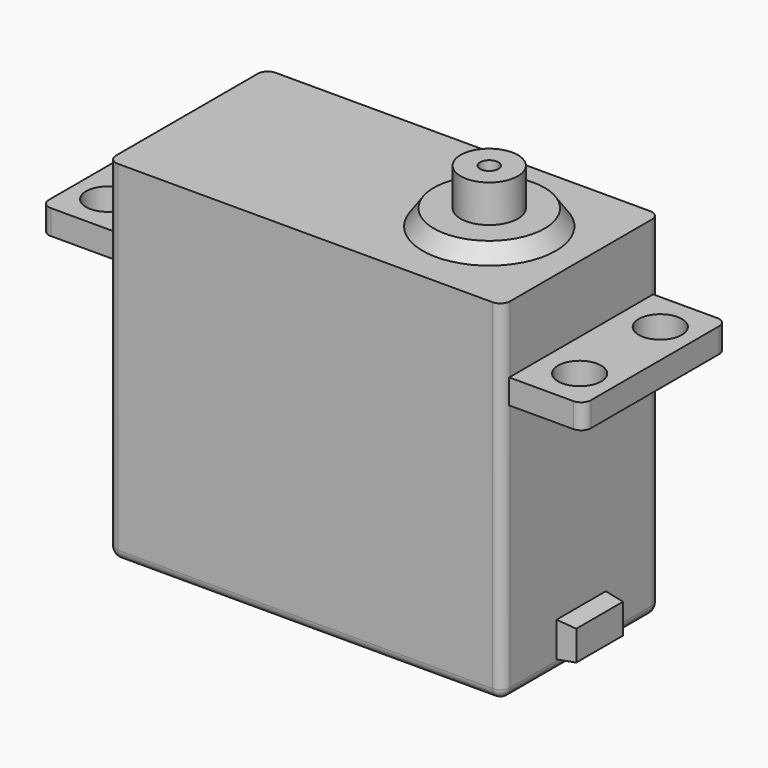
from build123d import *

# Parameters (mm, degrees)
F0_W           = 40.64
F0_H           = 20.32
F1_DEPTH       = 36.068
F2_W           = 6.35
F2_H           = 3.6068
F4_W           = 6.0198
F4_H           = 3.0734
F7_R           = 2.2225
F8_DEPTH       = 2.54
F9_R           = 6.858
F11_R          = 5.7023
F13_T1_DEPTH   = 38.608
F13_T3_DEPTH   = 18.288
F13_S7_W       = 1.016
F13_S7_H       = 1.016
F13_T8_DEPTH   = 1.016
F13_S13_W      = 1.016
F13_S13_H      = 1.016
F13_T14_DEPTH  = 1.016
F13_S19_W      = 1.016
F13_S19_H      = 1.016
F13_T20_DEPTH  = 1.016
F13_S25_W      = 1.016
F13_S25_H      = 1.016
F13_T26_DEPTH  = 1.016
F13_T32_DEPTH  = 37.592
F13_T38_DEPTH  = 37.592
F13_T44_DEPTH  = 37.592
F13_T51_DEPTH  = 37.592
F13_T57_DEPTH  = 37.592
F13_T63_DEPTH  = 37.592
F13_T69_DEPTH  = 37.592
F13_T75_DEPTH  = 37.592
F13_T82_DEPTH  = 37.592
F13_T88_DEPTH  = 37.592
F13_T94_DEPTH  = 37.592
F13_T100_DEPTH = 37.592
F13_T106_DEPTH = 37.592
F13_T113_DEPTH = 37.592
F13_T119_DEPTH = 37.592
F13_T125_DEPTH = 37.592
F13_T131_DEPTH = 37.592
F13_T137_DEPTH = 37.592
F13_T144_DEPTH = 37.592
F13_T150_DEPTH = 37.592
F14_R          = 2.95275
F14_R_2        = 0.9398
F15_DEPTH      = 3.8608


# Not quite as in the source:
# - a fillet or chamfer that OpenCascade refuses, or shapes differently, is made with other operations: its cross-section is extruded or revolved along the edge and cut away or added


with BuildPart() as f1:
    # F0 (on Top) → F1 (new body)
    with BuildSketch(Plane.XY):
        Rectangle(F0_W, F0_H)
    extrude(amount=F1_DEPTH)

    # F2 (on face) → F5 section 0
    with BuildSketch(Plane.YZ.offset(20.32)):
        with Locations((0, 2.9464)):
            Rectangle(F2_W, F2_H)
    # F4 (on offset) → F5 section 1
    with BuildSketch(Plane.YZ.offset(22.225)):
        with Locations((0, 2.9464)):
            Rectangle(F4_W, F4_H)
    loft()

    # F7 (on offset) → F8 (join)
    with BuildSketch(Plane.XY.offset(29.21)):
        with BuildLine():
            ThreePointArc((-27.94, -8.255), (-27.6424204897, -8.9734204897), (-26.924, -9.271))
            Line((-26.924, -9.271), (-20.32, -9.271))
            Line((-20.32, -9.271), (-20.32, 9.271))
            Line((-20.32, 9.271), (-26.924, 9.271))
            ThreePointArc((-26.924, 9.271), (-27.6424204897, 8.9734204897), (-27.94, 8.255))
            Line((-27.94, 8.255), (-27.94, -8.255))
        make_face()
        with Locations((-24.3205, -5.1943)):
            Circle(F7_R, mode=Mode.SUBTRACT)
        with Locations((-24.3205, 5.1943)):
            Circle(F7_R, mode=Mode.SUBTRACT)
        with BuildLine():
            ThreePointArc((27.94, 8.255), (27.6424204897, 8.9734204897), (26.924, 9.271))
            Line((26.924, 9.271), (20.32, 9.271))
            Line((20.32, 9.271), (20.32, -9.271))
            Line((20.32, -9.271), (26.924, -9.271))
            ThreePointArc((26.924, -9.271), (27.6424204897, -8.9734204897), (27.94, -8.255))
            Line((27.94, -8.255), (27.94, 8.255))
        make_face()
        with Locations((24.3205, -5.1943)):
            Circle(F7_R, mode=Mode.SUBTRACT)
        with Locations((24.3205, 5.1943)):
            Circle(F7_R, mode=Mode.SUBTRACT)
    extrude(amount=-F8_DEPTH)

    # F9 (on face) → F12 section 0
    with BuildSketch(Plane.XY.offset(36.068)):
        with Locations((10.8458, 0)):
            Circle(F9_R)
    # F11 (on offset) → F12 section 1
    with BuildSketch(Plane.XY.offset(37.719)):
        with Locations((10.8458, 0)):
            Circle(F11_R)
    loft()

    # F13: fillet of radius 1.016 on 8 edges, made by hand

    # F13_s2 → F13_t1 (cut)
    with BuildSketch(Plane.YZ.offset(-19.304)):
        with BuildLine():
            ThreePointArc((-10.16, 1.016), (-9.8624204897, 0.2975795103), (-9.144, 0))
            Line((-9.144, 0), (-10.16, 0))
            Line((-10.16, 0), (-10.16, 1.016))
        make_face()
        with BuildLine():
            ThreePointArc((9.144, 0), (9.8624204897, 0.2975795103), (10.16, 1.016))
            Line((10.16, 1.016), (10.16, 0))
            Line((10.16, 0), (9.144, 0))
        make_face()
    extrude(amount=F13_T1_DEPTH, mode=Mode.SUBTRACT)

    # F13_s4 → F13_t3 (cut)
    with BuildSketch(Plane.XZ.offset(-9.144)):
        with BuildLine():
            ThreePointArc((20.32, 1.016), (20.0224204897, 0.2975795103), (19.304, 0))
            Line((19.304, 0), (20.32, 0))
            Line((20.32, 0), (20.32, 1.016))
        make_face()
        with BuildLine():
            ThreePointArc((-19.304, 0), (-20.0224204897, 0.2975795103), (-20.32, 1.016))
            Line((-20.32, 1.016), (-20.32, 0))
            Line((-20.32, 0), (-19.304, 0))
        make_face()
    extrude(amount=F13_T3_DEPTH, mode=Mode.SUBTRACT)


with BuildPart() as f13_tool6:
    # F13_s7 → F13_t8 (new body)
    with BuildSketch(Plane.YZ.offset(19.304)):
        with Locations((-9.652, 0.508)):
            Rectangle(F13_S7_W, F13_S7_H)
    extrude(amount=F13_T8_DEPTH)

    # F13_s9 → F13_t10 (revolve, cut)
    with BuildSketch(Plane(origin=(19.304, -9.144, 1.016), x_dir=(0, 0.7071067812, 0.7071067812), z_dir=(0, 0.7071067812, -0.7071067812))):
        with BuildLine():
            ThreePointArc((0, -1.016), (1.016, 0), (0, 1.016))
            Line((0, 1.016), (0, -1.016))
        make_face()
    revolve(axis=Axis((19.304, -9.144, 1.016), (1, 0, 0)), mode=Mode.SUBTRACT)


with BuildPart() as f1_1:
    add(f1.part)

    # F13_t5: cut F13_tool6
    add(f13_tool6.part, mode=Mode.SUBTRACT)


with BuildPart() as f13_tool12:
    # F13_s13 → F13_t14 (new body)
    with BuildSketch(Plane.YZ.offset(19.304)):
        with Locations((9.652, 0.508)):
            Rectangle(F13_S13_W, F13_S13_H)
    extrude(amount=F13_T14_DEPTH)

    # F13_s15 → F13_t16 (revolve, cut)
    with BuildSketch(Plane(origin=(19.304, 9.144, 1.016), x_dir=(0, -0.7071067812, 0.7071067812), z_dir=(0, 0.7071067812, 0.7071067812))):
        with BuildLine():
            ThreePointArc((0, -1.016), (1.016, 0), (0, 1.016))
            Line((0, 1.016), (0, -1.016))
        make_face()
    revolve(axis=Axis((19.304, 9.144, 1.016), (1, 0, 0)), mode=Mode.SUBTRACT)


with BuildPart() as f1_2:
    add(f1_1.part)

    # F13_t11: cut F13_tool12
    add(f13_tool12.part, mode=Mode.SUBTRACT)


with BuildPart() as f13_tool18:
    # F13_s19 → F13_t20 (new body)
    with BuildSketch(Plane.XY.offset(1.016)):
        with Locations((-19.812, 9.652)):
            Rectangle(F13_S19_W, F13_S19_H)
    extrude(amount=-F13_T20_DEPTH)

    # F13_s21 → F13_t22 (revolve, cut)
    with BuildSketch(Plane(origin=(-19.304, 9.144, 1.016), x_dir=(0.7071067812, -0.7071067812, 0), z_dir=(0.7071067812, 0.7071067812, 0))):
        with BuildLine():
            ThreePointArc((0, -1.016), (1.016, 0), (0, 1.016))
            Line((0, 1.016), (0, -1.016))
        make_face()
    revolve(axis=Axis((-19.304, 9.144, 1.016), (0, 0, -1)), mode=Mode.SUBTRACT)


with BuildPart() as f1_3:
    add(f1_2.part)

    # F13_t17: cut F13_tool18
    add(f13_tool18.part, mode=Mode.SUBTRACT)


with BuildPart() as f13_tool24:
    # F13_s25 → F13_t26 (new body)
    with BuildSketch(Plane.XZ.offset(9.144)):
        with Locations((-19.812, 0.508)):
            Rectangle(F13_S25_W, F13_S25_H)
    extrude(amount=F13_T26_DEPTH)

    # F13_s27 → F13_t28 (revolve, cut)
    with BuildSketch(Plane(origin=(-19.304, -9.144, 1.016), x_dir=(0.7071067812, 0, 0.7071067812), z_dir=(0.7071067812, 0, -0.7071067812))):
        with BuildLine():
            ThreePointArc((0, -1.016), (1.016, 0), (0, 1.016))
            Line((0, 1.016), (0, -1.016))
        make_face()
    revolve(axis=Axis((-19.304, -9.144, 1.016), (0, -1, 0)), mode=Mode.SUBTRACT)


with BuildPart() as f1_4:
    add(f1_3.part)

    # F13_t23: cut F13_tool24
    add(f13_tool24.part, mode=Mode.SUBTRACT)


with BuildPart() as f13_tool30:
    # F13_s31 → F13_t32 (new body)
    with BuildSketch(Plane.XY.offset(1.016)):
        with BuildLine():
            ThreePointArc((20.32, -9.144), (20.0224204897, -9.8624204897), (19.304, -10.16))
            Line((19.304, -10.16), (20.32, -10.16))
            Line((20.32, -10.16), (20.32, -9.144))
        make_face()
    extrude(amount=F13_T32_DEPTH)

    split(bisect_by=Plane.XY.offset(26.67), keep=Keep.BOTTOM)

    split(bisect_by=Plane.XZ.offset(9.271), keep=Keep.BOTTOM)


with BuildPart() as f1_5:
    add(f1_4.part)

    # F13_t29: cut F13_tool30
    add(f13_tool30.part, mode=Mode.SUBTRACT)


with BuildPart() as f13_tool36:
    # F13_s37 → F13_t38 (new body)
    with BuildSketch(Plane.XY.offset(1.016)):
        with BuildLine():
            ThreePointArc((20.32, -9.144), (20.0224204897, -9.8624204897), (19.304, -10.16))
            Line((19.304, -10.16), (20.32, -10.16))
            Line((20.32, -10.16), (20.32, -9.144))
        make_face()
    extrude(amount=F13_T38_DEPTH)

    split(bisect_by=Plane.XY.offset(26.67), keep=Keep.BOTTOM)

    split(bisect_by=Plane.XZ.offset(9.271), keep=Keep.TOP)


with BuildPart() as f1_6:
    add(f1_5.part)

    # F13_t35: cut F13_tool36
    add(f13_tool36.part, mode=Mode.SUBTRACT)


with BuildPart() as f13_tool42:
    # F13_s43 → F13_t44 (new body)
    with BuildSketch(Plane.XY.offset(1.016)):
        with BuildLine():
            ThreePointArc((20.32, -9.144), (20.0224204897, -9.8624204897), (19.304, -10.16))
            Line((19.304, -10.16), (20.32, -10.16))
            Line((20.32, -10.16), (20.32, -9.144))
        make_face()
    extrude(amount=F13_T44_DEPTH)

    split(bisect_by=Plane.XY.offset(26.67), keep=Keep.TOP)

    split(bisect_by=Plane.XZ.offset(9.271), keep=Keep.TOP)

    split(bisect_by=Plane.XY.offset(29.21), keep=Keep.BOTTOM)


with BuildPart() as f1_7:
    add(f1_6.part)

    # F13_t41: cut F13_tool42
    add(f13_tool42.part, mode=Mode.SUBTRACT)


with BuildPart() as f13_tool49:
    # F13_s50 → F13_t51 (new body)
    with BuildSketch(Plane.XY.offset(1.016)):
        with BuildLine():
            ThreePointArc((20.32, -9.144), (20.0224204897, -9.8624204897), (19.304, -10.16))
            Line((19.304, -10.16), (20.32, -10.16))
            Line((20.32, -10.16), (20.32, -9.144))
        make_face()
    extrude(amount=F13_T51_DEPTH)

    split(bisect_by=Plane.XZ.offset(9.271), keep=Keep.BOTTOM)

    split(bisect_by=Plane.XY.offset(29.21), keep=Keep.TOP)


with BuildPart() as f1_8:
    add(f1_7.part)

    # F13_t48: cut F13_tool49
    add(f13_tool49.part, mode=Mode.SUBTRACT)


with BuildPart() as f13_tool55:
    # F13_s56 → F13_t57 (new body)
    with BuildSketch(Plane.XY.offset(1.016)):
        with BuildLine():
            ThreePointArc((20.32, -9.144), (20.0224204897, -9.8624204897), (19.304, -10.16))
            Line((19.304, -10.16), (20.32, -10.16))
            Line((20.32, -10.16), (20.32, -9.144))
        make_face()
    extrude(amount=F13_T57_DEPTH)

    split(bisect_by=Plane.XZ.offset(9.271), keep=Keep.TOP)

    split(bisect_by=Plane.XY.offset(29.21), keep=Keep.TOP)


with BuildPart() as f1_9:
    add(f1_8.part)

    # F13_t54: cut F13_tool55
    add(f13_tool55.part, mode=Mode.SUBTRACT)


with BuildPart() as f13_tool61:
    # F13_s62 → F13_t63 (new body)
    with BuildSketch(Plane.XY.offset(1.016)):
        with BuildLine():
            ThreePointArc((20.32, 9.144), (20.0224204897, 9.8624204897), (19.304, 10.16))
            Line((19.304, 10.16), (20.32, 10.16))
            Line((20.32, 10.16), (20.32, 9.144))
        make_face()
    extrude(amount=F13_T63_DEPTH)

    split(bisect_by=Plane.XZ.offset(-9.271), keep=Keep.TOP)

    split(bisect_by=Plane.XY.offset(26.67), keep=Keep.BOTTOM)


with BuildPart() as f1_10:
    add(f1_9.part)

    # F13_t60: cut F13_tool61
    add(f13_tool61.part, mode=Mode.SUBTRACT)


with BuildPart() as f13_tool67:
    # F13_s68 → F13_t69 (new body)
    with BuildSketch(Plane.XY.offset(1.016)):
        with BuildLine():
            ThreePointArc((20.32, 9.144), (20.0224204897, 9.8624204897), (19.304, 10.16))
            Line((19.304, 10.16), (20.32, 10.16))
            Line((20.32, 10.16), (20.32, 9.144))
        make_face()
    extrude(amount=F13_T69_DEPTH)

    split(bisect_by=Plane.XZ.offset(-9.271), keep=Keep.BOTTOM)

    split(bisect_by=Plane.XY.offset(26.67), keep=Keep.BOTTOM)


with BuildPart() as f1_11:
    add(f1_10.part)

    # F13_t66: cut F13_tool67
    add(f13_tool67.part, mode=Mode.SUBTRACT)


with BuildPart() as f13_tool73:
    # F13_s74 → F13_t75 (new body)
    with BuildSketch(Plane.XY.offset(1.016)):
        with BuildLine():
            ThreePointArc((20.32, 9.144), (20.0224204897, 9.8624204897), (19.304, 10.16))
            Line((19.304, 10.16), (20.32, 10.16))
            Line((20.32, 10.16), (20.32, 9.144))
        make_face()
    extrude(amount=F13_T75_DEPTH)

    split(bisect_by=Plane.XZ.offset(-9.271), keep=Keep.BOTTOM)

    split(bisect_by=Plane.XY.offset(26.67), keep=Keep.TOP)

    split(bisect_by=Plane.XY.offset(29.21), keep=Keep.BOTTOM)


with BuildPart() as f1_12:
    add(f1_11.part)

    # F13_t72: cut F13_tool73
    add(f13_tool73.part, mode=Mode.SUBTRACT)


with BuildPart() as f13_tool80:
    # F13_s81 → F13_t82 (new body)
    with BuildSketch(Plane.XY.offset(1.016)):
        with BuildLine():
            ThreePointArc((20.32, 9.144), (20.0224204897, 9.8624204897), (19.304, 10.16))
            Line((19.304, 10.16), (20.32, 10.16))
            Line((20.32, 10.16), (20.32, 9.144))
        make_face()
    extrude(amount=F13_T82_DEPTH)

    split(bisect_by=Plane.XZ.offset(-9.271), keep=Keep.TOP)

    split(bisect_by=Plane.XY.offset(29.21), keep=Keep.TOP)


with BuildPart() as f1_13:
    add(f1_12.part)

    # F13_t79: cut F13_tool80
    add(f13_tool80.part, mode=Mode.SUBTRACT)


with BuildPart() as f13_tool86:
    # F13_s87 → F13_t88 (new body)
    with BuildSketch(Plane.XY.offset(1.016)):
        with BuildLine():
            ThreePointArc((20.32, 9.144), (20.0224204897, 9.8624204897), (19.304, 10.16))
            Line((19.304, 10.16), (20.32, 10.16))
            Line((20.32, 10.16), (20.32, 9.144))
        make_face()
    extrude(amount=F13_T88_DEPTH)

    split(bisect_by=Plane.XZ.offset(-9.271), keep=Keep.BOTTOM)

    split(bisect_by=Plane.XY.offset(29.21), keep=Keep.TOP)


with BuildPart() as f1_14:
    add(f1_13.part)

    # F13_t85: cut F13_tool86
    add(f13_tool86.part, mode=Mode.SUBTRACT)


with BuildPart() as f13_tool92:
    # F13_s93 → F13_t94 (new body)
    with BuildSketch(Plane.XY.offset(1.016)):
        with BuildLine():
            ThreePointArc((-19.304, 10.16), (-20.0224204897, 9.8624204897), (-20.32, 9.144))
            Line((-20.32, 9.144), (-20.32, 10.16))
            Line((-20.32, 10.16), (-19.304, 10.16))
        make_face()
    extrude(amount=F13_T94_DEPTH)

    split(bisect_by=Plane.XY.offset(26.67), keep=Keep.BOTTOM)

    split(bisect_by=Plane.XZ.offset(-9.271), keep=Keep.BOTTOM)


with BuildPart() as f1_15:
    add(f1_14.part)

    # F13_t91: cut F13_tool92
    add(f13_tool92.part, mode=Mode.SUBTRACT)


with BuildPart() as f13_tool98:
    # F13_s99 → F13_t100 (new body)
    with BuildSketch(Plane.XY.offset(1.016)):
        with BuildLine():
            ThreePointArc((-19.304, 10.16), (-20.0224204897, 9.8624204897), (-20.32, 9.144))
            Line((-20.32, 9.144), (-20.32, 10.16))
            Line((-20.32, 10.16), (-19.304, 10.16))
        make_face()
    extrude(amount=F13_T100_DEPTH)

    split(bisect_by=Plane.XY.offset(26.67), keep=Keep.BOTTOM)

    split(bisect_by=Plane.XZ.offset(-9.271), keep=Keep.TOP)


with BuildPart() as f1_16:
    add(f1_15.part)

    # F13_t97: cut F13_tool98
    add(f13_tool98.part, mode=Mode.SUBTRACT)


with BuildPart() as f13_tool104:
    # F13_s105 → F13_t106 (new body)
    with BuildSketch(Plane.XY.offset(1.016)):
        with BuildLine():
            ThreePointArc((-19.304, 10.16), (-20.0224204897, 9.8624204897), (-20.32, 9.144))
            Line((-20.32, 9.144), (-20.32, 10.16))
            Line((-20.32, 10.16), (-19.304, 10.16))
        make_face()
    extrude(amount=F13_T106_DEPTH)

    split(bisect_by=Plane.XY.offset(26.67), keep=Keep.TOP)

    split(bisect_by=Plane.XZ.offset(-9.271), keep=Keep.BOTTOM)

    split(bisect_by=Plane.XY.offset(29.21), keep=Keep.BOTTOM)


with BuildPart() as f1_17:
    add(f1_16.part)

    # F13_t103: cut F13_tool104
    add(f13_tool104.part, mode=Mode.SUBTRACT)


with BuildPart() as f13_tool111:
    # F13_s112 → F13_t113 (new body)
    with BuildSketch(Plane.XY.offset(1.016)):
        with BuildLine():
            ThreePointArc((-19.304, 10.16), (-20.0224204897, 9.8624204897), (-20.32, 9.144))
            Line((-20.32, 9.144), (-20.32, 10.16))
            Line((-20.32, 10.16), (-19.304, 10.16))
        make_face()
    extrude(amount=F13_T113_DEPTH)

    split(bisect_by=Plane.XZ.offset(-9.271), keep=Keep.BOTTOM)

    split(bisect_by=Plane.XY.offset(29.21), keep=Keep.TOP)


with BuildPart() as f1_18:
    add(f1_17.part)

    # F13_t110: cut F13_tool111
    add(f13_tool111.part, mode=Mode.SUBTRACT)


with BuildPart() as f13_tool117:
    # F13_s118 → F13_t119 (new body)
    with BuildSketch(Plane.XY.offset(1.016)):
        with BuildLine():
            ThreePointArc((-19.304, 10.16), (-20.0224204897, 9.8624204897), (-20.32, 9.144))
            Line((-20.32, 9.144), (-20.32, 10.16))
            Line((-20.32, 10.16), (-19.304, 10.16))
        make_face()
    extrude(amount=F13_T119_DEPTH)

    split(bisect_by=Plane.XZ.offset(-9.271), keep=Keep.TOP)

    split(bisect_by=Plane.XY.offset(29.21), keep=Keep.TOP)


with BuildPart() as f1_19:
    add(f1_18.part)

    # F13_t116: cut F13_tool117
    add(f13_tool117.part, mode=Mode.SUBTRACT)


with BuildPart() as f13_tool123:
    # F13_s124 → F13_t125 (new body)
    with BuildSketch(Plane.XY.offset(1.016)):
        with BuildLine():
            ThreePointArc((-19.304, -10.16), (-20.0224204897, -9.8624204897), (-20.32, -9.144))
            Line((-20.32, -9.144), (-20.32, -10.16))
            Line((-20.32, -10.16), (-19.304, -10.16))
        make_face()
    extrude(amount=F13_T125_DEPTH)

    split(bisect_by=Plane.XZ.offset(9.271), keep=Keep.TOP)

    split(bisect_by=Plane.XY.offset(26.67), keep=Keep.BOTTOM)


with BuildPart() as f1_20:
    add(f1_19.part)

    # F13_t122: cut F13_tool123
    add(f13_tool123.part, mode=Mode.SUBTRACT)


with BuildPart() as f13_tool129:
    # F13_s130 → F13_t131 (new body)
    with BuildSketch(Plane.XY.offset(1.016)):
        with BuildLine():
            ThreePointArc((-19.304, -10.16), (-20.0224204897, -9.8624204897), (-20.32, -9.144))
            Line((-20.32, -9.144), (-20.32, -10.16))
            Line((-20.32, -10.16), (-19.304, -10.16))
        make_face()
    extrude(amount=F13_T131_DEPTH)

    split(bisect_by=Plane.XZ.offset(9.271), keep=Keep.BOTTOM)

    split(bisect_by=Plane.XY.offset(26.67), keep=Keep.BOTTOM)


with BuildPart() as f1_21:
    add(f1_20.part)

    # F13_t128: cut F13_tool129
    add(f13_tool129.part, mode=Mode.SUBTRACT)


with BuildPart() as f13_tool135:
    # F13_s136 → F13_t137 (new body)
    with BuildSketch(Plane.XY.offset(1.016)):
        with BuildLine():
            ThreePointArc((-19.304, -10.16), (-20.0224204897, -9.8624204897), (-20.32, -9.144))
            Line((-20.32, -9.144), (-20.32, -10.16))
            Line((-20.32, -10.16), (-19.304, -10.16))
        make_face()
    extrude(amount=F13_T137_DEPTH)

    split(bisect_by=Plane.XZ.offset(9.271), keep=Keep.TOP)

    split(bisect_by=Plane.XY.offset(26.67), keep=Keep.TOP)

    split(bisect_by=Plane.XY.offset(29.21), keep=Keep.BOTTOM)


with BuildPart() as f1_22:
    add(f1_21.part)

    # F13_t134: cut F13_tool135
    add(f13_tool135.part, mode=Mode.SUBTRACT)


with BuildPart() as f13_tool142:
    # F13_s143 → F13_t144 (new body)
    with BuildSketch(Plane.XY.offset(1.016)):
        with BuildLine():
            ThreePointArc((-19.304, -10.16), (-20.0224204897, -9.8624204897), (-20.32, -9.144))
            Line((-20.32, -9.144), (-20.32, -10.16))
            Line((-20.32, -10.16), (-19.304, -10.16))
        make_face()
    extrude(amount=F13_T144_DEPTH)

    split(bisect_by=Plane.XZ.offset(9.271), keep=Keep.TOP)

    split(bisect_by=Plane.XY.offset(29.21), keep=Keep.TOP)


with BuildPart() as f1_23:
    add(f1_22.part)

    # F13_t141: cut F13_tool142
    add(f13_tool142.part, mode=Mode.SUBTRACT)


with BuildPart() as f13_tool148:
    # F13_s149 → F13_t150 (new body)
    with BuildSketch(Plane.XY.offset(1.016)):
        with BuildLine():
            ThreePointArc((-19.304, -10.16), (-20.0224204897, -9.8624204897), (-20.32, -9.144))
            Line((-20.32, -9.144), (-20.32, -10.16))
            Line((-20.32, -10.16), (-19.304, -10.16))
        make_face()
    extrude(amount=F13_T150_DEPTH)

    split(bisect_by=Plane.XZ.offset(9.271), keep=Keep.BOTTOM)

    split(bisect_by=Plane.XY.offset(29.21), keep=Keep.TOP)


with BuildPart() as f1_24:
    add(f1_23.part)

    # F13_t147: cut F13_tool148
    add(f13_tool148.part, mode=Mode.SUBTRACT)

    # F14 (on face) → F15 (join)
    with BuildSketch(Plane.XY.offset(37.719)):
        with Locations((10.8458, 0)):
            Circle(F14_R)
        with Locations((10.8458, 0)):
            Circle(F14_R_2, mode=Mode.SUBTRACT)
    extrude(amount=F15_DEPTH)


solid = f1_24.part
